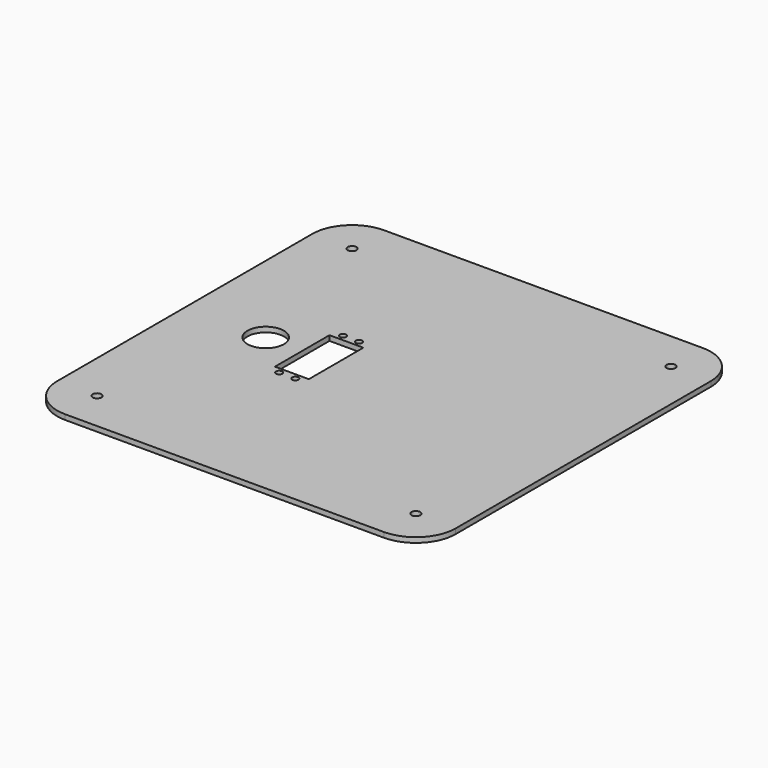
from build123d import *

# Parameters (mm, degrees)
F0_R     = 2.7608867496
F0_R_2   = 2
F0_W     = 21.25
F0_H     = 42.75
F0_R_3   = 11.43
F1_DEPTH = 3.175


# Not quite as in the source:
# - a length typed as a fraction of an inch, garbled in the dataset ("3 / 203.2 mm" for 3/8 in), is restored


with BuildPart() as f1:
    # F0 (on Top) → F1 (new body)
    with BuildSketch(Plane.XY):
        with BuildLine():
            Line((100, 126.1928240007), (-100, 126.1928240007))
            ThreePointArc((-100, 126.1928240007), (-117.6776695297, 118.8704935303), (-125, 101.1928240007))
            Line((-125, 101.1928240007), (-125, -98.8071759993))
            ThreePointArc((-125, -98.8071759993), (-117.6776695297, -116.484845529), (-100, -123.8071759993))
            Line((-100, -123.8071759993), (100, -123.8071759993))
            ThreePointArc((100, -123.8071759993), (117.6776695297, -116.484845529), (125, -98.8071759993))
            Line((125, -98.8071759993), (125, 101.1928240007))
            ThreePointArc((125, 101.1928240007), (117.6776695297, 118.8704935303), (100, 126.1928240007))
        make_face()
        with Locations((-100, -98.8071759993)):
            Circle(F0_R, mode=Mode.SUBTRACT)
        with Locations((-45.7576233894, -23.8071759993)):
            Circle(F0_R_2, mode=Mode.SUBTRACT)
        with Locations((-35.6076233894, -23.8071759993)):
            Circle(F0_R_2, mode=Mode.SUBTRACT)
        with Locations((-40.6826233894, 1.1928240007)):
            Rectangle(F0_W, F0_H, mode=Mode.SUBTRACT)
        with Locations((100, -98.8071759993)):
            Circle(F0_R, mode=Mode.SUBTRACT)
        with Locations((-74.2, 1.1928240007)):
            Circle(F0_R_3, mode=Mode.SUBTRACT)
        with Locations((-45.7576233894, 26.1928240007)):
            Circle(F0_R_2, mode=Mode.SUBTRACT)
        with Locations((-35.6076233894, 26.1928240007)):
            Circle(F0_R_2, mode=Mode.SUBTRACT)
        with Locations((-100, 101.1928240007)):
            Circle(F0_R, mode=Mode.SUBTRACT)
        with Locations((100, 101.1928240007)):
            Circle(F0_R, mode=Mode.SUBTRACT)
    extrude(amount=F1_DEPTH)


solid = f1.part
